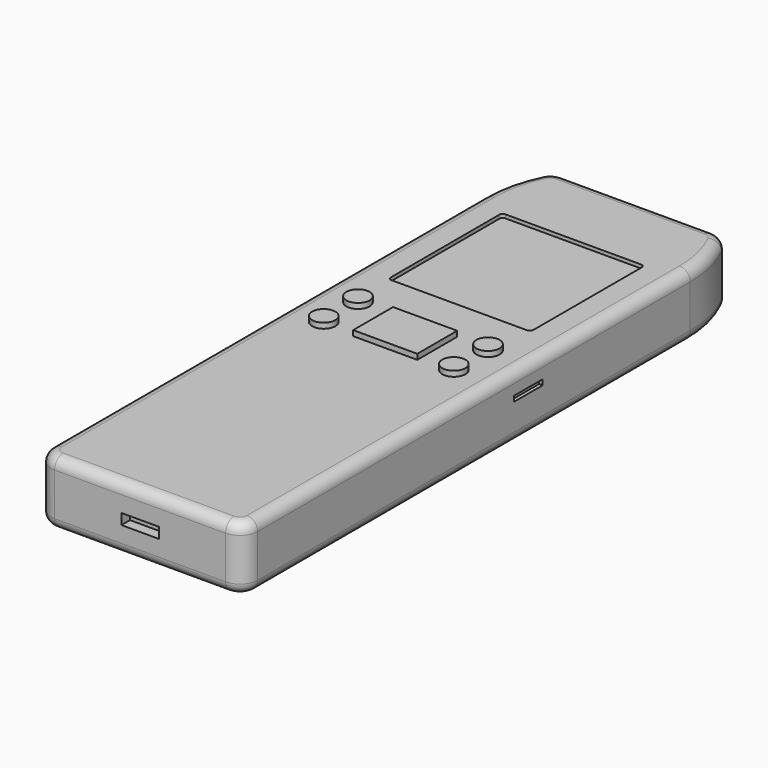
from build123d import *

# Parameters (mm, degrees)
F0_W        = 58
F0_H        = 175
F1_DEPTH    = 18
F2_SIZE2    = 10
F2_SIZE     = 5
F3_R        = 5
F4_T1_DEPTH = 59.306306
F6_DEPTH    = 1
F5_R        = 3.25
F5_W        = 18
F5_H        = 14
F7_DEPTH    = 1.5
F8_W        = 2
F8_H        = 6
F9_DEPTH    = 1
F10_R       = 3
F11_R       = 0.99999
F12_W       = 10.5
F12_H       = 3
F13_DEPTH   = 3
F14_W       = 10
F14_H       = 1.5
F15_DEPTH   = 1
F16_W       = 10
F16_H       = 1.5
F17_DEPTH   = 1


# Not quite as in the source:
# - a fillet or chamfer that OpenCascade refuses, or shapes differently, is made with other operations: its cross-section is extruded or revolved along the edge and cut away or added
# - a fillet or chamfer is up to 0.001 mm smaller than in the source, because OpenCascade refuses the exact size


with BuildPart() as f1:
    # F0 (on Top) → F1 (new body)
    with BuildSketch(Plane.XY):
        with Locations((29, 87.5)):
            Rectangle(F0_W, F0_H)
    extrude(amount=F1_DEPTH)

    # F2
    f2_edges = [f1.edges().sort_by_distance(p)[0] for p in [
        (58, 175, 9),
        (0, 175, 9),
    ]]
    f2_side = f1.faces().sort_by_distance((29, 175, 9))[0]
    chamfer(f2_edges, length=F2_SIZE, length2=F2_SIZE2, reference=f2_side)

    # F3
    f3_edges = [f1.edges().sort_by_distance(p)[0] for p in [
        (0, 0, 9),
        (58, 0, 9),
        (5, 175, 9),
        (53, 175, 9),
    ]]
    fillet(f3_edges, radius=F3_R)

    # F4: fillet of radius 35 on 2 edges, made by hand

    # F4_s2 → F4_t1 (cut)
    with BuildSketch(Plane.XY.offset(-20.653153)):
        with BuildLine():
            ThreePointArc((0, 156.738739), (0.913213, 164.681721), (3.605198, 172.21021))
            Line((3.605198, 172.21021), (0.465718, 173.757357))
            ThreePointArc((0.465718, 173.757357), (0.487539, 173.801316), (-3.130495, 166.565248))
            Line((-3.130495, 166.565248), (-3.5, 165))
            Line((-3.5, 165), (-3.5, 156.738739))
            Line((-3.5, 156.738739), (0, 156.738739))
        make_face()
        with BuildLine():
            ThreePointArc((58, 156.738739), (57.086787, 164.681721), (54.394802, 172.21021))
            Line((54.394802, 172.21021), (57.534282, 173.757357))
            ThreePointArc((57.534282, 173.757357), (57.512461, 173.801316), (61.130495, 166.565248))
            Line((61.130495, 166.565248), (61.5, 165))
            Line((61.5, 165), (61.5, 156.738739))
            Line((61.5, 156.738739), (58, 156.738739))
        make_face()
    extrude(amount=F4_T1_DEPTH, mode=Mode.SUBTRACT)

    # F5 (on face) → F6 (cut)
    with BuildSketch(Plane.XY.offset(18)):
        with BuildLine():
            Line((48, 152), (10, 152))
            ThreePointArc((10, 152), (9.292893, 151.707107), (9, 151))
            Line((9, 151), (9, 113))
            ThreePointArc((9, 113), (9.292893, 112.292893), (10, 112))
            Line((10, 112), (48, 112))
            ThreePointArc((48, 112), (48.707107, 112.292893), (49, 113))
            Line((49, 113), (49, 151))
            ThreePointArc((49, 151), (48.707107, 151.707107), (48, 152))
        make_face()
    extrude(amount=-F6_DEPTH, mode=Mode.SUBTRACT)

    # F5 (on face) → F7 (join)
    with BuildSketch(Plane.XY.offset(18)):
        with Locations((47.25, 99.25)):
            Circle(F5_R)
        with Locations((29, 93)):
            Rectangle(F5_W, F5_H)
        with Locations((10.75, 99.25)):
            Circle(F5_R)
        with Locations((10.75, 87.25)):
            Circle(F5_R)
        with Locations((47.25, 87.25)):
            Circle(F5_R)
    extrude(amount=F7_DEPTH)

    # F8 (on face) → F9 (join)
    with BuildSketch(Plane(origin=(0, 0, 0), x_dir=(1, 0, 0), z_dir=(0, 0, -1))):
        with Locations((6, -31)):
            Rectangle(F8_W, F8_H)
        with Locations((52, -31)):
            Rectangle(F8_W, F8_H)
        with Locations((52, -132)):
            Rectangle(F8_W, F8_H)
        with Locations((6, -132)):
            Rectangle(F8_W, F8_H)
    extrude(amount=F9_DEPTH)

    # F10 (call 1 of 4: OpenCascade refuses the feature's edges together)
    f10_edges = [f1.edges().sort_by_distance(p)[0] for p in [
        (58, 80.869369, 18),
    ]]
    fillet(f10_edges, radius=F10_R)

    # F10#2 (call 2 of 4)
    f10_2_edges = [f1.edges().sort_by_distance(p)[0] for p in [
        (58, 80.869369, 0),
    ]]
    fillet(f10_2_edges, radius=F10_R)

    # F10#3 (call 3 of 4)
    f10_3_edges = [f1.edges().sort_by_distance(p)[0] for p in [
        (29, 175, 18),
    ]]
    fillet(f10_3_edges, radius=F10_R)

    # F10#4 (call 4 of 4)
    f10_4_edges = [f1.edges().sort_by_distance(p)[0] for p in [
        (29, 175, 0),
    ]]
    fillet(f10_4_edges, radius=F10_R)

    # F11 (radius 1 in the source; OpenCascade refuses exactly that, so slightly less here)
    f11_edges = [f1.edges().sort_by_distance(p)[0] for p in [
        (52, 34, -1),
        (52, 28, -1),
        (6, 28, -1),
        (6, 34, -1),
        (6, 129, -1),
        (6, 135, -1),
        (52, 129, -1),
        (52, 135, -1),
    ]]
    fillet(f11_edges, radius=F11_R)

    # F12 (on face) → F13 (cut)
    with BuildSketch(Plane.XZ):
        with Locations((29, 9)):
            Rectangle(F12_W, F12_H)
    extrude(amount=-F13_DEPTH, mode=Mode.SUBTRACT)

    # F14 (on face) → F15 (cut)
    with BuildSketch(Plane.YZ.offset(58)):
        with Locations((100, 11.25)):
            Rectangle(F14_W, F14_H)
    extrude(amount=-F15_DEPTH, mode=Mode.SUBTRACT)

    # F16 (on face) → F17 (cut)
    with BuildSketch(Plane(origin=(0, 0, 0), x_dir=(0, -1, 0), z_dir=(-1, 0, 0))):
        with Locations((-100, 11.25)):
            Rectangle(F16_W, F16_H)
    extrude(amount=-F17_DEPTH, mode=Mode.SUBTRACT)


solid = f1.part
